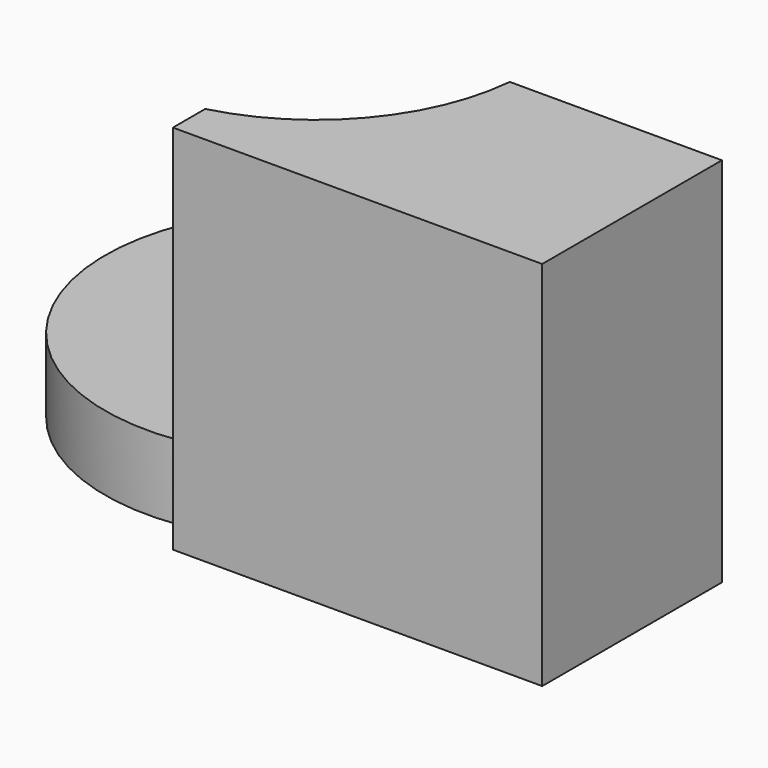
from build123d import *

# Parameters (mm, degrees)
F1_DEPTH    = 25.4
F2_DEPTH    = 5.08
F3_T4_ANGLE = 174.1930400009


# Not quite as in the source:
# - a fillet or chamfer that OpenCascade refuses, or shapes differently, is made with other operations: its cross-section is extruded or revolved along the edge and cut away or added


with BuildPart() as f1:
    # F0 (on Top) → F1 (new body)
    with BuildSketch(Plane.XY):
        with BuildLine():
            Line((-28.7617053837, 23.086078465), (-43.2633440317, 23.086078465))
            ThreePointArc((-43.2633440317, 23.086078465), (-46.6420182582, 15.0906140017), (-54.0029779077, 10.4907048123))
            Line((-54.0029779077, 10.4907048123), (-54.0029779077, 7.7324733138))
            Line((-54.0029779077, 7.7324733138), (-28.7617053837, 7.7324733138))
            Line((-28.7617053837, 7.7324733138), (-28.7617053837, 23.086078465))
        make_face()
    extrude(amount=F1_DEPTH)

    # F0 (on Top) → F2 (join)
    with BuildSketch(Plane.XY):
        with BuildLine():
            Line((-54.0029779077, 10.4907048123), (-54.0029779077, 23.086078465))
            Line((-54.0029779077, 23.086078465), (-43.2633440317, 23.086078465))
            ThreePointArc((-43.2633440317, 23.086078465), (-43.2161007803, 23.7580355867), (-43.2003415292, 24.4314670563))
            ThreePointArc((-43.2003415292, 24.4314670563), (-68.9767505511, 33.249655712), (-54.0029779077, 10.4907048123))
        make_face()
        with BuildLine():
            Line((-43.2633440317, 23.086078465), (-54.0029779077, 23.086078465))
            Line((-54.0029779077, 23.086078465), (-54.0029779077, 10.4907048123))
            ThreePointArc((-54.0029779077, 10.4907048123), (-46.6420182582, 15.0906140017), (-43.2633440317, 23.086078465))
        make_face()
    extrude(amount=F2_DEPTH)

    # F3: chamfer of 5.08 on 1 edges, made by hand


with BuildPart() as f3_tool2:
    # F3_s3 → F3_t4 (revolve)
    with BuildSketch(Plane(origin=(-48.0088326829, 36.9045281739, 0), x_dir=(0, 0, 1), z_dir=(-0.7928262046, 0.6094477905, 0))):
        Polygon((10.16, -30.128971911), (5.08, -25.048971911), (5.08, -30.128971911), align=None)
    revolve(axis=Axis((-57.5969107449, 24.4314670563, 5.08), (0, 0, 1)), revolution_arc=F3_T4_ANGLE)

    split(bisect_by=Plane.XZ.offset(-23.086078465), keep=Keep.TOP)

    split(bisect_by=Plane.YZ.offset(-54.0029779077), keep=Keep.TOP)


with BuildPart() as f1_1:
    add(f1.part)

    # F3_t1: union F3_tool2
    add(f3_tool2.part)


solid = f1_1.part
